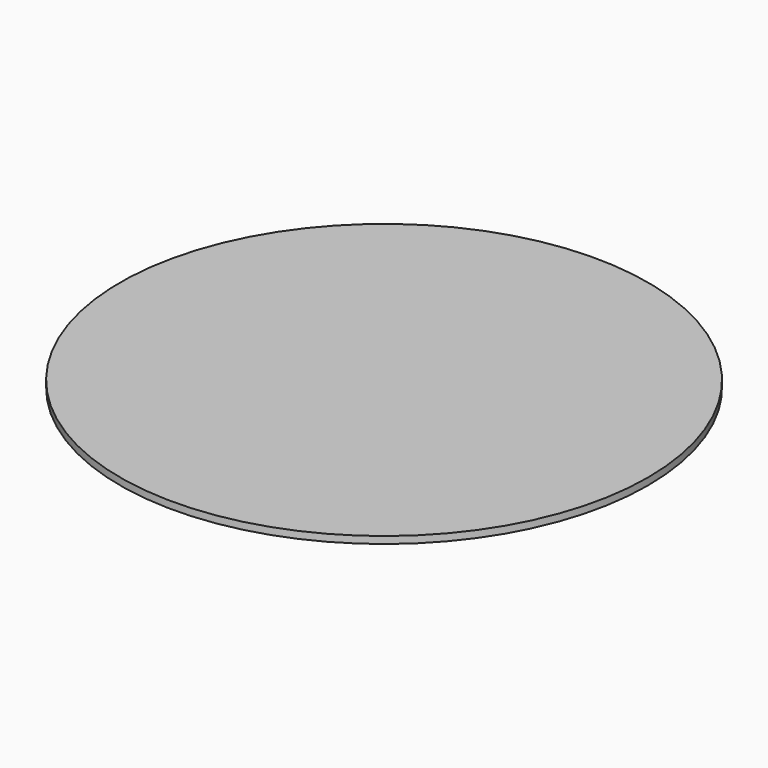
from build123d import *

# Parameters (mm, degrees)
F1_R     = 19.05
F3_DEPTH = 0.508


# Not quite as in the source:
# - the program builds the solid bodies; features that only make, move or delete a surface that nothing else refers to are left out


with BuildPart() as f3:
    # F1 (on Top) → F3 (new body)
    with BuildSketch(Plane.XY):
        Circle(F1_R)
    extrude(amount=F3_DEPTH)


solid = f3.part
